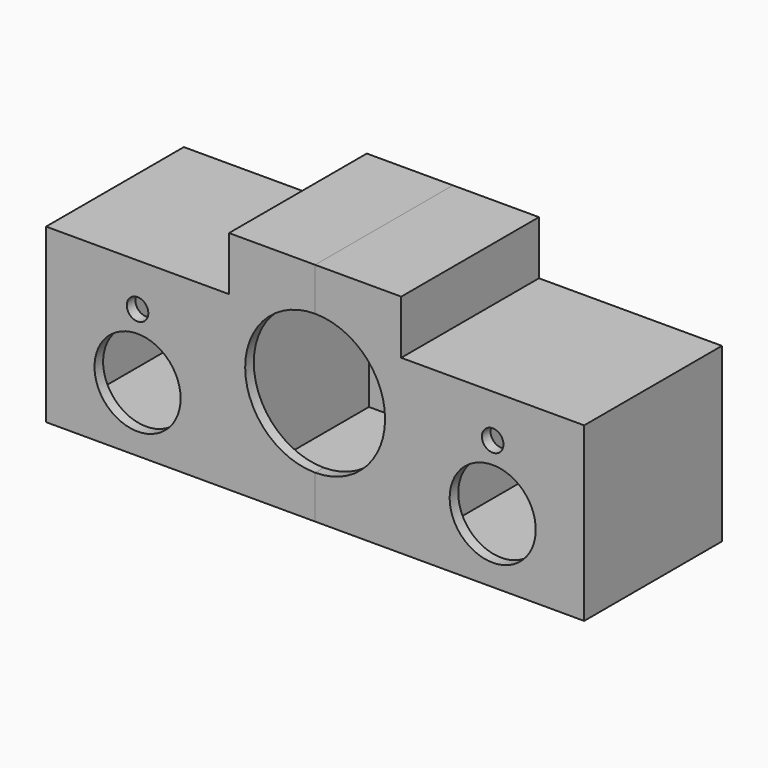
from build123d import *
from build123d import SkipClean  # not in build123d's __all__

# Parameters (mm, degrees)
F0_W      = 203.2
F0_H      = 203.2
F1_DEPTH  = 12.7
F2_W      = 203.2
F2_H      = 203.2
F2_W_2    = 177.8
F2_H_2    = 177.8
F3_DEPTH  = 254
F4_W      = 203.2
F4_H      = 203.2
F4_W_2    = 177.8
F4_H_2    = 177.8
F5_DEPTH  = 12.7
F6_W      = 203.2
F6_H      = 203.2
F7_DEPTH  = 12.7
F8_W      = 203.2
F8_H      = 203.2
F8_W_2    = 177.8
F8_H_2    = 177.8
F9_DEPTH  = 203.2
F10_W     = 12.7
F10_H     = 177.8
F11_DEPTH = 177.8
F12_R     = 50.8
F12_R_2   = 12.7
F12_R_3   = 82.55
F13_DEPTH = 25.4
F15_DEPTH = 203.2


with BuildPart() as f1:
    # F0 (on Top) → F1 (new body)
    with BuildSketch(Plane.XY):
        Rectangle(F0_W, F0_H)
    extrude(amount=F1_DEPTH)

    # F2 (on face) → F3 (join)
    with BuildSketch(Plane.XY.offset(12.7)):
        Rectangle(F2_W, F2_H)
        Rectangle(F2_W_2, F2_H_2, mode=Mode.SUBTRACT)
    extrude(amount=F3_DEPTH)

    # F4 (on face) → F5 (join)
    with BuildSketch(Plane.XY.offset(266.7)):
        Rectangle(F4_W, F4_H)
        Rectangle(F4_W_2, F4_H_2, mode=Mode.SUBTRACT)
        Rectangle(F4_W_2, F4_H_2)
    extrude(amount=-F5_DEPTH)

    # F6 (on face) → F7 (join)
    with BuildSketch(Plane(origin=(-101.6, 0, 0), x_dir=(0, -1, 0), z_dir=(-1, 0, 0))):
        with Locations((0, 101.6)):
            Rectangle(F6_W, F6_H)
    extrude(amount=F7_DEPTH)

    # F8 (on face) → F9 (join)
    with BuildSketch(Plane(origin=(-114.3, 0, 0), x_dir=(0, -1, 0), z_dir=(-1, 0, 0))):
        with Locations((0, 101.6)):
            Rectangle(F8_W, F8_H)
        with Locations((0, 101.6)):
            Rectangle(F8_W_2, F8_H_2, mode=Mode.SUBTRACT)
    extrude(amount=F9_DEPTH)

    # F10 (on face) → F11 (join)
    with BuildSketch(Plane.XY.offset(12.7)):
        with Locations((-311.15, 0)):
            Rectangle(F10_W, F10_H)
    extrude(amount=F11_DEPTH)

    # F12 (on face) → F13 (cut)
    with BuildSketch(Plane.XZ.offset(101.6)):
        with Locations((-209.55, 76.2)):
            Circle(F12_R)
        with Locations((-209.55, 152.4)):
            Circle(F12_R_2)
        with Locations((0, 133.35)):
            Circle(F12_R_3)
    extrude(amount=-F13_DEPTH, mode=Mode.SUBTRACT)

    # F14 (on face) → F15 (cut)
    with BuildSketch(Plane.XZ.offset(101.6)):
        with BuildLine():
            Line((101.6, 0), (101.6, 266.7))
            Line((101.6, 266.7), (0, 266.7))
            Line((0, 266.7), (0, 215.9))
            ThreePointArc((0, 215.9), (58.3716647869, 191.7216647869), (82.55, 133.35))
            ThreePointArc((82.55, 133.35), (58.3716647869, 74.9783352131), (0, 50.8))
            Line((0, 50.8), (0, 0))
            Line((0, 0), (101.6, 0))
        make_face()
        with BuildLine():
            ThreePointArc((82.55, 133.35), (58.3716647869, 191.7216647869), (0, 215.9))
            Line((0, 215.9), (0, 50.8))
            ThreePointArc((0, 50.8), (58.3716647869, 74.9783352131), (82.55, 133.35))
        make_face()
    extrude(amount=-F15_DEPTH, mode=Mode.SUBTRACT)

    # F16: F1 across face


with BuildPart() as f1_1:
    add(f1.part, clean=False)
    with SkipClean():  # cleaning this boolean's faces spoils the solid; the shape is the same uncleaned
        add(f1.part.mirror(Plane(origin=(0, 21.7236842105, 133.35), x_dir=(0, 1, 0), z_dir=(1, 0, 0))), clean=False)


solid = f1_1.part
